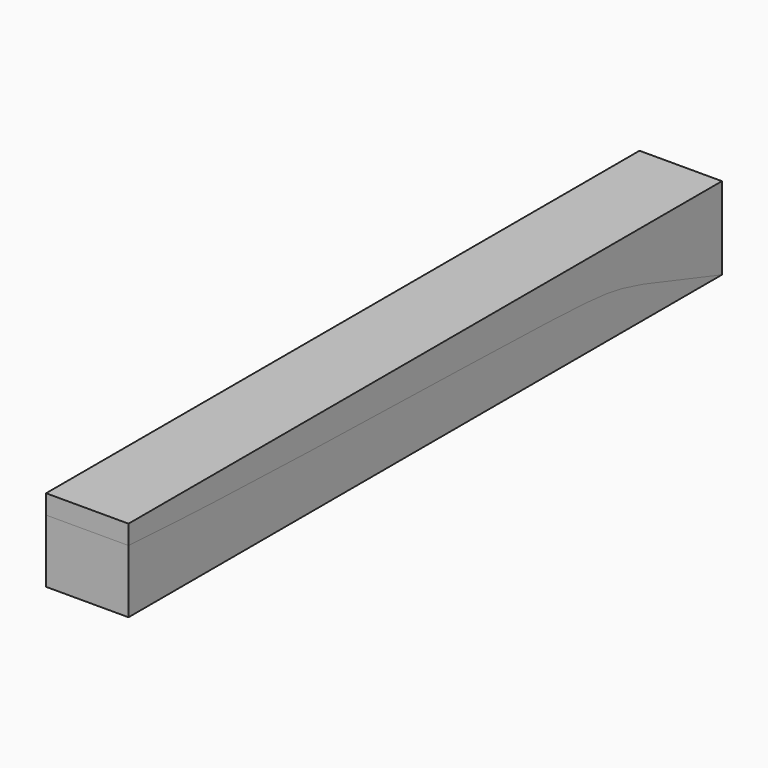
from build123d import *

# Parameters (mm, degrees)
F0_W     = 10
F0_H     = 90
F1_DEPTH = 10
F3_DEPTH = 10
F4_W     = 5
F4_H     = 5
F5_DEPTH = 25


with BuildPart() as f1:
    # F0 (on Top) → F1 (new body)
    with BuildSketch(Plane.XY):
        Rectangle(F0_W, F0_H)
    extrude(amount=F1_DEPTH)


with BuildPart() as f3:
    # F2 (on face) → F3 (new body)
    with BuildSketch(Plane(origin=(-5, 0, 0), x_dir=(0, -1, 0), z_dir=(-1, 0, 0))):
        with BuildLine():
            add(Edge.make_bspline(
                [(-45, 0), (-30.9047084302, 4.547316581), (-29.684083025, 5.9774667313), (24.6960557997, 6.3660335727), (45, 7.6651168056)],
                knots=[0, 0, 0, 0, 0.366960811, 1, 1, 1, 1], degree=3))
            Line((-45, 0), (45, 0))
            Line((45, 0), (45, 7.6651168056))
        make_face()
    extrude(amount=-F3_DEPTH)

    # F4 (on face) → F5 (join)
    with BuildSketch(Plane(origin=(0, 45, 0), x_dir=(-1, 0, 0), z_dir=(0, 1, 0))):
        with Locations((2.5, 2.5)):
            Rectangle(F4_W, F4_H)
    extrude(amount=-F5_DEPTH)


solid = Compound([f1.part, f3.part])
